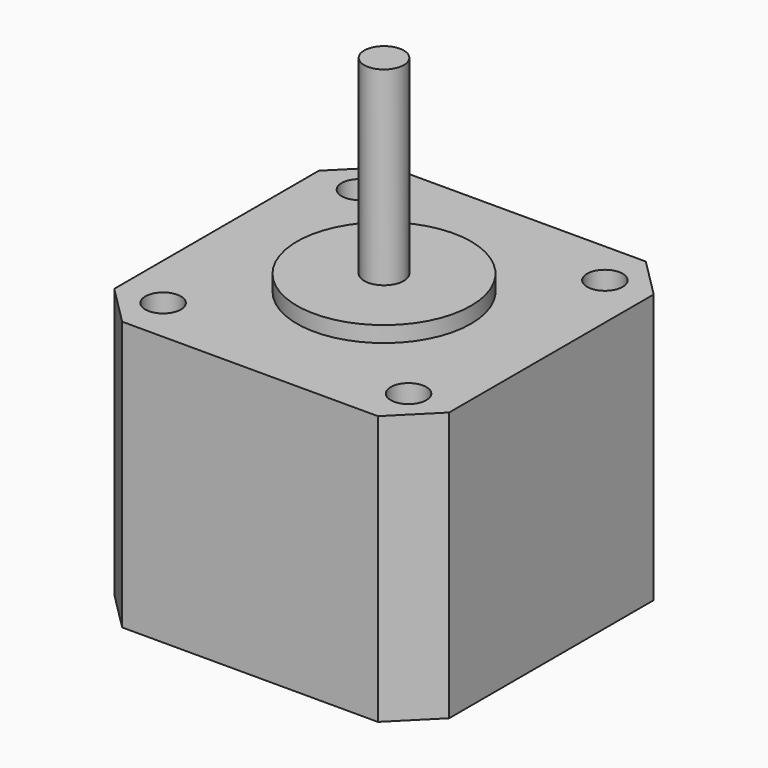
from build123d import *

# Parameters (mm, degrees)
F0_W            = 42.3
F0_H            = 42.3
F1_DEPTH        = 34
F2_R            = 11
F3_DEPTH        = 2
F4_R            = 2.5
F5_DEPTH        = 24
F6_R            = 2.25
F7_DEPTH        = 5
F7_COPIES_COUNT = 4
F8_SIZE         = 5


# Not quite as in the source:
# - a pattern or mirror of a feature is missing from the dataset's text; its kind, count and spacing are read off the source's solid


with BuildPart() as f1:
    # F0 (on Top) → F1 (new body)
    with BuildSketch(Plane.XY):
        Rectangle(F0_W, F0_H)
    extrude(amount=F1_DEPTH)

    # F2 (on face) → F3 (join)
    with BuildSketch(Plane.XY.offset(34)):
        Circle(F2_R)
    extrude(amount=F3_DEPTH)

    # F4 (on face) → F5 (join)
    with BuildSketch(Plane.XY.offset(36)):
        Circle(F4_R)
    extrude(amount=F5_DEPTH)

    # F6 (on face) → F7 (cut)
    with BuildSketch(Plane.XY.offset(34)):
        with Locations((-15.5, 15.5)):
            Circle(F6_R)
    f7 = extrude(amount=-F7_DEPTH, mode=Mode.SUBTRACT)

    # F7_copies: F7 ×4 about axis
    f7_copies_axis = Axis((0, 0, 0), (0, 0, 1))
    for i in range(1, F7_COPIES_COUNT):
        add(f7.rotate(f7_copies_axis, i * 360 / F7_COPIES_COUNT), mode=Mode.SUBTRACT)

    # F8
    f8_edges = [f1.edges().sort_by_distance(p)[0] for p in [
        (-21.15, -21.15, 17),
        (-21.15, 21.15, 17),
        (21.15, 21.15, 17),
        (21.15, -21.15, 17),
    ]]
    chamfer(f8_edges, length=F8_SIZE)


solid = f1.part
